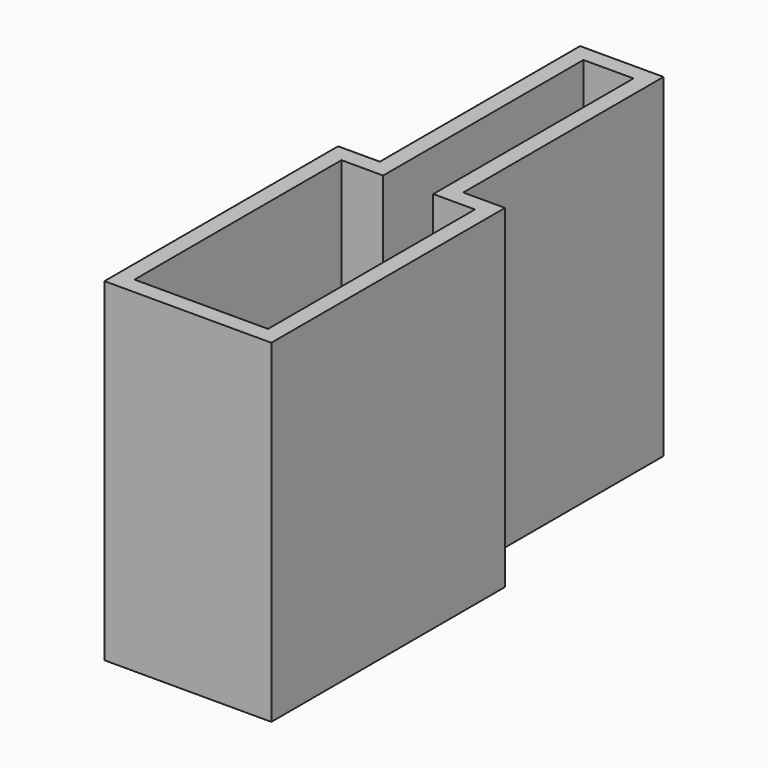
from build123d import *

# Parameters (mm, degrees)
F1_DEPTH = 50.8
F2_T     = -2.54


with BuildPart() as f1:
    # F0 (on Top) → F1 (new body)
    with BuildSketch(Plane.XY):
        Polygon((0, 44.45), (0, 0), (25.4, 0), (25.4, 44.45), (19.05, 44.45), (19.05, 82.55), (6.35, 82.55), (6.35, 44.45), align=None)
    extrude(amount=F1_DEPTH)

    # F2
    f2_openings = [f1.faces().sort_by_distance(p)[0] for p in [
        (12.7, 34.6075, 50.8),
    ]]
    offset(amount=F2_T, openings=f2_openings, kind=Kind.INTERSECTION)


solid = f1.part
